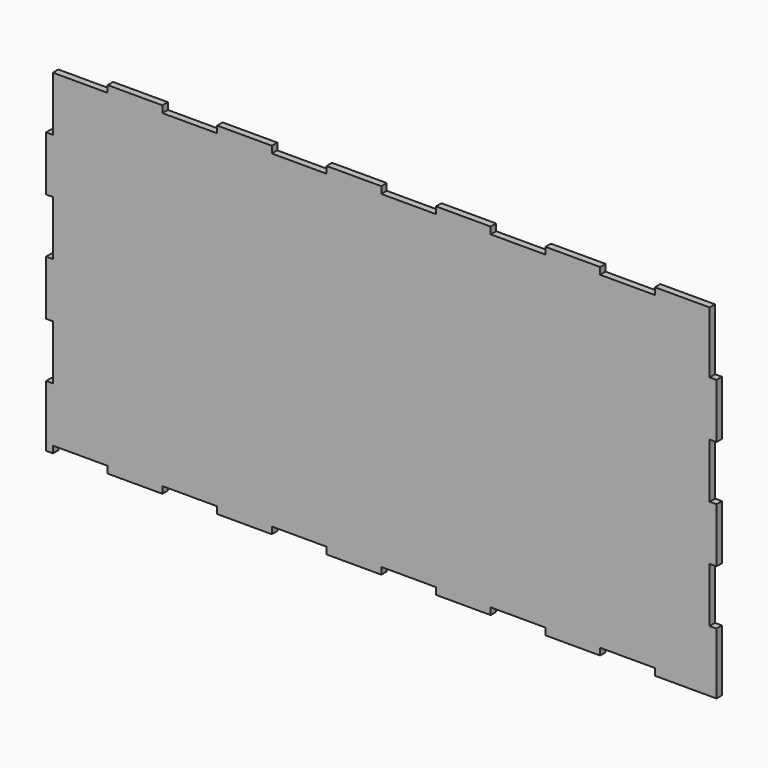
from build123d import *

# Parameters (mm, degrees)
F1_DEPTH = 3.175


# Not quite as in the source:
# - a length typed as a fraction of an inch, garbled in the dataset ("3 / 203.2 mm" for 3/8 in), is restored


with BuildPart() as f1:
    # F0 (on Front) → F1 (new body)
    with BuildSketch(Plane.XZ):
        Polygon((-178.9622853069, -44.2643848114), (-153.5622853069, -44.2643848114), (-153.5622853069, -47.4393848114), (-128.1622853069, -47.4393848114), (-128.1622853069, -44.2643848114), (-102.7622853069, -44.2643848114), (-102.7622853069, -47.4393848114), (-77.3622853069, -47.4393848114), (-77.3622853069, -44.2643848114), (-51.9622853069, -44.2643848114), (-51.9622853069, -47.4393848114), (-26.5622853069, -47.4393848114), (-26.5622853069, -44.2643848114), (-26.5622853069, 108.1356151886), (-26.5622853069, 111.3106151886), (-51.9622853069, 111.3106151886), (-51.9622853069, 108.1356151886), (-77.3622853069, 108.1356151886), (-77.3622853069, 111.3106151886), (-102.7622853069, 111.3106151886), (-102.7622853069, 108.1356151886), (-128.1622853069, 108.1356151886), (-128.1622853069, 111.3106151886), (-153.5622853069, 111.3106151886), (-153.5622853069, 108.1356151886), (-178.9622853069, 108.1356151886), (-178.9622853069, 82.7356151886), (-182.1372853069, 82.7356151886), (-182.1372853069, 57.3356151886), (-178.9622853069, 57.3356151886), (-178.9622853069, 31.9356151886), (-182.1372853069, 31.9356151886), (-182.1372853069, 6.5356151886), (-178.9622853069, 6.5356151886), (-178.9622853069, -18.8643848114), (-182.1372853069, -18.8643848114), (-182.1372853069, -44.2643848114), (-182.1372853069, -47.4393848114), (-178.9622853069, -47.4393848114), align=None)
        Polygon((-26.5622853069, 108.1356151886), (-26.5622853069, -44.2643848114), (-1.1622853069, -44.2643848114), (-1.1622853069, -47.4393848114), (24.2377146931, -47.4393848114), (24.2377146931, -44.2643848114), (49.6377146931, -44.2643848114), (49.6377146931, -47.4393848114), (75.0377146931, -47.4393848114), (75.0377146931, -44.2643848114), (100.4377146931, -44.2643848114), (100.4377146931, -47.4393848114), (125.8377146931, -47.4393848114), (129.0127146931, -47.4393848114), (129.0127146931, -44.2643848114), (129.0127146931, -18.8643848114), (125.8377146931, -18.8643848114), (125.8377146931, 6.5356151886), (129.0127146931, 6.5356151886), (129.0127146931, 31.9356151886), (125.8377146931, 31.9356151886), (125.8377146931, 57.3356151886), (129.0127146931, 57.3356151886), (129.0127146931, 82.7356151886), (125.8377146931, 82.7356151886), (125.8377146931, 108.1356151886), (125.8377146931, 111.3106151886), (100.4377146931, 111.3106151886), (100.4377146931, 108.1356151886), (75.0377146931, 108.1356151886), (75.0377146931, 111.3106151886), (49.6377146931, 111.3106151886), (49.6377146931, 108.1356151886), (24.2377146931, 108.1356151886), (24.2377146931, 111.3106151886), (-1.1622853069, 111.3106151886), (-1.1622853069, 108.1356151886), align=None)
    extrude(amount=F1_DEPTH)


solid = f1.part
